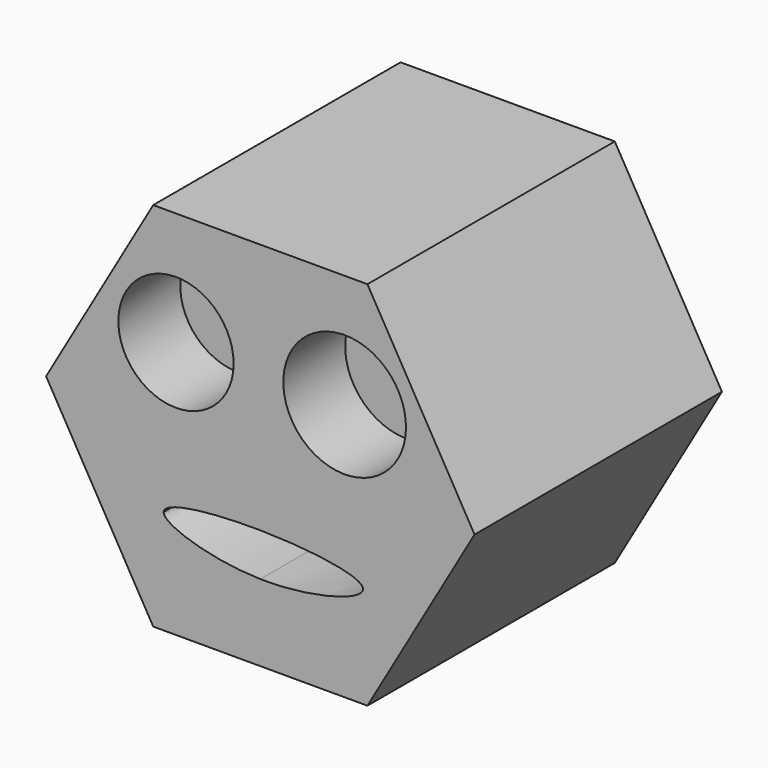
from build123d import *

# Parameters (mm, degrees)
F1_DEPTH = 20
F2_R     = 3.9672544226
F2_R_2   = 3.7268973953
F4_DEPTH = 5
F6_R     = 4.0640636786
F7_DEPTH = 5
F8_DEPTH = 5


# Not quite as in the source:
# - the program builds the solid bodies; features that only make, move or delete a surface that nothing else refers to are left out


with BuildPart() as f1:
    # F0 (on Front) → F1 (new body)
    with BuildSketch(Plane.XZ):
        Polygon((-6.9287490553, -12.0009453967), (6.9287490553, -12.0009453967), (13.8574981107, 0), (6.9287490553, 12.0009453967), (-6.9287490553, 12.0009453967), (-13.8574981107, 0), align=None)
    extrude(amount=F1_DEPTH)

    # F2 (on face) → F4 (cut)
    with BuildSketch(Plane.XZ.offset(20)):
        with Locations((5.454974249, 4.6615242027)):
            Circle(F2_R)
        with Locations((-5.4549747147, 4.6615242027)):
            Circle(F2_R_2)
    extrude(amount=-F4_DEPTH, mode=Mode.SUBTRACT)

    # F6 (on face) → F7 (cut)
    with BuildSketch(Plane(origin=(0, 0, -12.0009453967), x_dir=(1, 0, 0), z_dir=(0, 0, -1))):
        with Locations((0, 9.6756508574)):
            Circle(F6_R)
    extrude(amount=-F7_DEPTH, mode=Mode.SUBTRACT)

    # F3 (on face) → F8 (cut)
    with BuildSketch(Plane.XZ.offset(20)):
        with BuildLine():
            Line((0, -5.3527420043), (0, -7.04187667))
            add(Edge.make_bspline(
                [(6.6451518796, -5.4549751803), (6.6575654316, -6.1571957747), (3.2728013866, -7.1077153996), (0, -7.04187667)],
                knots=[0.7456529131, 0.7456529131, 0.7456529131, 0.7456529131, 1, 1, 1, 1], degree=3))
            Line((6.6451518796, -5.4549751803), (0, -5.3527420043))
        make_face()
        with BuildLine():
            Line((0, -5.3527420043), (6.6451518796, -5.4549751803))
            add(Edge.make_bspline(
                [(0, -4.2647989467), (3.2636275259, -4.3042470372), (6.6328122368, -4.7569355417), (6.6451518796, -5.4549751803)],
                knots=[0.492820185, 0.492820185, 0.492820185, 0.492820185, 0.7456529131, 0.7456529131, 0.7456529131, 0.7456529131], degree=3))
            Line((0, -4.2647989467), (0, -5.3527420043))
        make_face()
        with BuildLine():
            add(Edge.make_bspline(
                [(-6.2484252267, -5.2566123195), (-6.2199094707, -4.57569338), (-3.1594165925, -4.2266104736), (0, -4.2647989467)],
                knots=[0.2480606621, 0.2480606621, 0.2480606621, 0.2480606621, 0.492820185, 0.492820185, 0.492820185, 0.492820185], degree=3))
            Line((-6.2484252267, -5.2566123195), (0, -5.3527420043))
            Line((0, -5.3527420043), (0, -4.2647989467))
        make_face()
        with BuildLine():
            add(Edge.make_bspline(
                [(0, -7.04187667), (-3.191911057, -6.9776652057), (-6.2773255825, -5.9467150004), (-6.2484252267, -5.2566123195)],
                knots=[0, 0, 0, 0, 0.2480606621, 0.2480606621, 0.2480606621, 0.2480606621], degree=3))
            Line((0, -7.04187667), (0, -5.3527420043))
            Line((0, -5.3527420043), (-6.2484252267, -5.2566123195))
        make_face()
    extrude(amount=-F8_DEPTH, mode=Mode.SUBTRACT)


solid = f1.part
